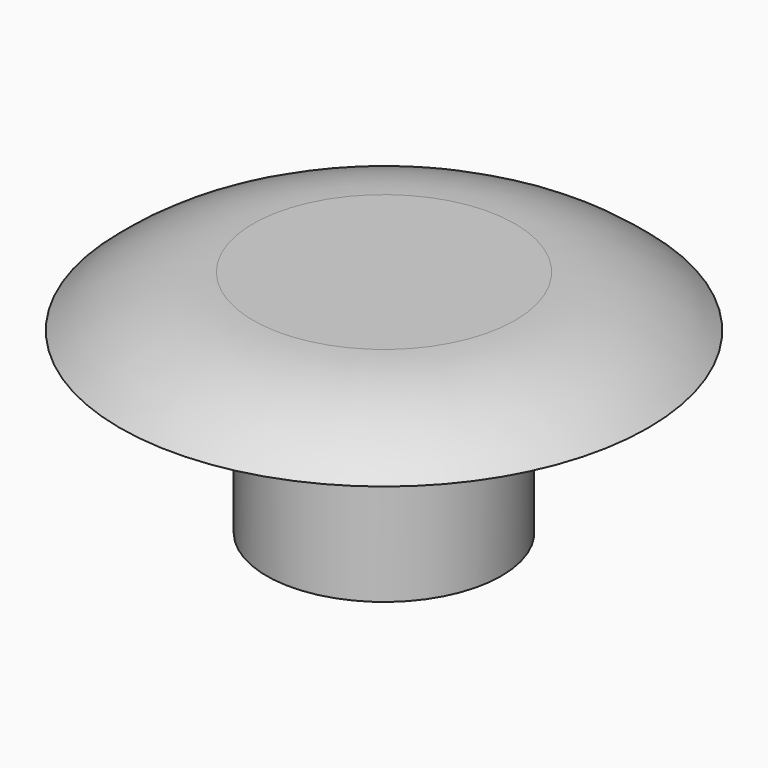
from build123d import *

# Parameters (mm, degrees)
F0_R     = 9.7995430213
F0_R_2   = 4.3563305412
F1_DEPTH = 1.905
F0_R_3   = 2.7204723389
F2_DEPTH = 1.905
F3_DEPTH = 6.604


# Not quite as in the source:
# - a fillet or chamfer that OpenCascade refuses, or shapes differently, is made with other operations: its cross-section is extruded or revolved along the edge and cut away or added


with BuildPart() as f1:
    # F0 (on Top) → F1 (new body)
    with BuildSketch(Plane.XY):
        Circle(F0_R)
        Circle(F0_R_2, mode=Mode.SUBTRACT)
    extrude(amount=F1_DEPTH)

    # F0 (on Top) → F2 (join)
    with BuildSketch(Plane.XY):
        Circle(F0_R_2)
        Circle(F0_R_3, mode=Mode.SUBTRACT)
        Circle(F0_R_3)
    extrude(amount=F2_DEPTH)

    # F0 (on Top) → F3 (join)
    with BuildSketch(Plane.XY):
        Circle(F0_R_2)
        Circle(F0_R_3, mode=Mode.SUBTRACT)
    extrude(amount=-F3_DEPTH)

    # F4: fillet of radius 7.3585229381 on 1 edges, made by hand

    # F4_s1 → F4_t2 (revolve, cut)
    with BuildSketch(Plane.XZ):
        with BuildLine():
            ThreePointArc((9.7995430213, 0), (7.5066545293, 1.4122520897), (4.8592042279, 1.905))
            Line((4.8592042279, 1.905), (9.7995430213, 1.905))
            Line((9.7995430213, 1.905), (9.7995430213, 0))
        make_face()
    revolve(axis=Axis((0, 0, 1.905), (0, 0, 1)), mode=Mode.SUBTRACT)


solid = f1.part
